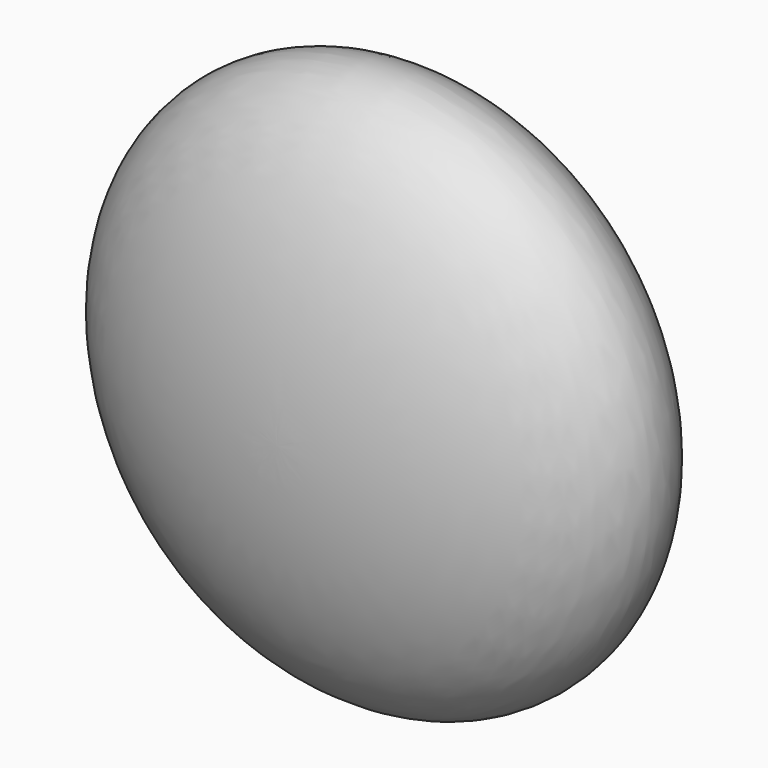
from build123d import *


# Not quite as in the source:
# - a feature of the source that left no trace in its solid (it failed there, or was rolled back) is left out


with BuildPart() as f8:
    # F7 (on Right) → F8 (revolve)
    with BuildSketch(Plane.YZ):
        with BuildLine():
            Line((8.6479444287, 0), (50.8378002562, 0))
            add(Edge.make_bspline(
                [(50.8378002562, 0), (50.8378002562, 43.8203215599), (29.7428723425, 43.8203215599), (8.6479444287, 43.8203215599), (8.6479444287, 0)],
                knots=[1.5707963268, 1.5707963268, 1.5707963268, 3.1415926536, 3.1415926536, 4.7123889804, 4.7123889804, 4.7123889804], degree=2, weights=[1, 0.7071067812, 1, 0.7071067812, 1]))
        make_face()
    revolve(axis=Axis((0, 34.41664204, 0), (0, 1, 0)))


solid = f8.part
